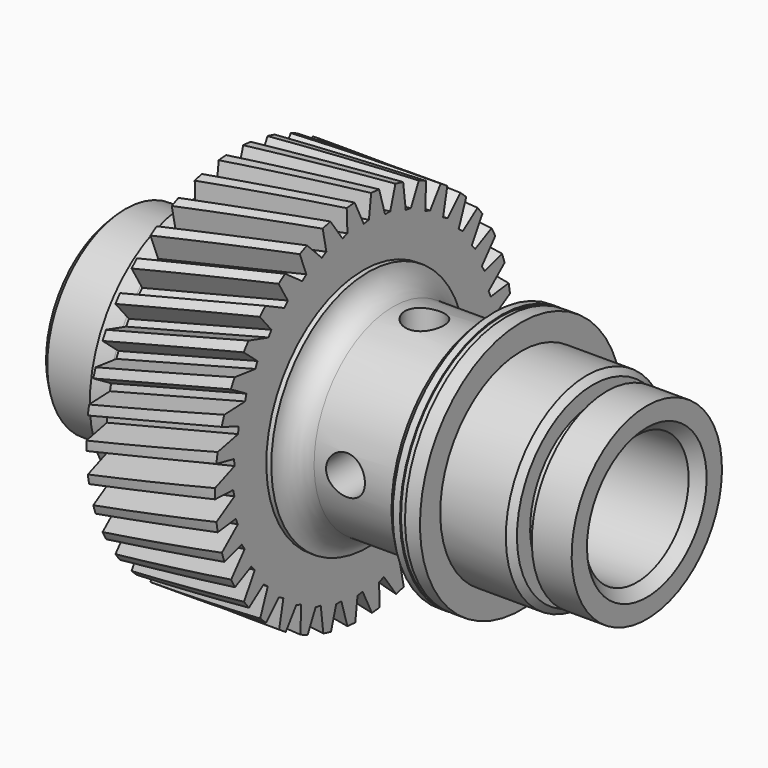
from build123d import *

# Parameters (mm, degrees)
F3_R             = 3.175
F4_SIZE          = 1.5748
F5_SIZE          = 2.54
F6_R             = 4.953
F7_DEPTH         = 47.2196
F7_DEPTH_BACK    = 47.2196
F8_R             = 4.953
F9_DEPTH         = 47.2196
F9_DEPTH_BACK    = 47.2196
F14_COPIES_COUNT = 38


# Not quite as in the source:
# - a fillet or chamfer that OpenCascade refuses, or shapes differently, is made with other operations: its cross-section is extruded or revolved along the edge and cut away or added
# - a pattern or mirror of a feature is missing from the dataset's text; its kind, count and spacing are read off the source's solid


with BuildPart() as f1:
    # F0 (on Front) → F1 (revolve)
    with BuildSketch(Plane.XZ):
        Polygon((0, 24.9174), (0, 18.6055), (28.575, 18.6055), (28.575, 13.4874), (99.4918, 13.4874), (99.4918, 16.51), (134.4168, 16.51), (134.4168, 23.9395), (124.2568, 23.9395), (124.2568, 20.0152), (120.7008, 20.0152), (120.7008, 25.7937), (102.4128, 25.7937), (102.4128, 32.258), (98.6028, 32.258), (98.6028, 31.9405), (97.3328, 31.9405), (97.3328, 32.258), (93.9038, 32.258), (93.9038, 25.146), (63.4238, 25.146), (63.4238, 30.8737), (62.1538, 30.8737), (62.1538, 47.2186), (29.3878, 47.2186), (29.3878, 32.258), (18.288, 32.258), (18.288, 24.9174), align=None)
    revolve(axis=Axis((67.2084, 0, 0), (1, 0, 0)))

    # F2: fillet of radius 6.35 on 2 edges, made by hand

    # F2_s1 → F2_t2 (revolve)
    with BuildSketch(Plane.XZ):
        with BuildLine():
            ThreePointArc((69.7432337333, 25.146), (65.4787938522, 26.7909970776), (63.4238, 30.8737))
            Line((63.4238, 30.8737), (63.4238, 25.146))
            Line((63.4238, 25.146), (69.7432337333, 25.146))
        make_face()
    revolve(axis=Axis((63.4238, 0, 0), (1, 0, 0)))

    # F2_s3 → F2_t4 (revolve)
    with BuildSketch(Plane.XZ):
        with BuildLine():
            ThreePointArc((29.3878, 38.608), (27.5279280605, 34.1178719395), (23.0378, 32.258))
            Line((23.0378, 32.258), (29.3878, 32.258))
            Line((29.3878, 32.258), (29.3878, 38.608))
        make_face()
    revolve(axis=Axis((29.3878, 0, 0), (1, 0, 0)))

    # F3
    f3_edges = [f1.edges().sort_by_distance(p)[0] for p in [
        (93.9038, 0, -25.146),
    ]]
    fillet(f3_edges, radius=F3_R)

    # F4
    f4_edges = [f1.edges().sort_by_distance(p)[0] for p in [
        (93.9038, 0, -32.258),
        (120.7008, 0, -25.7937),
        (0, 0, -24.9174),
    ]]
    chamfer(f4_edges, length=F4_SIZE)

    # F5
    f5_edges = [f1.edges().sort_by_distance(p)[0] for p in [
        (0, 0, -18.6055),
        (134.4168, 0, -16.51),
    ]]
    chamfer(f5_edges, length=F5_SIZE)

    # F6 (on Top) → F7 (cut, two sides)
    with BuildSketch(Plane.XY) as f7_sk:
        with Locations((77.7494, 0)):
            Circle(F6_R)
    extrude(amount=-F7_DEPTH, mode=Mode.SUBTRACT)
    extrude(f7_sk.sketch, amount=F7_DEPTH_BACK, mode=Mode.SUBTRACT)

    # F8 (on Front) → F9 (cut, two sides)
    with BuildSketch(Plane.XZ) as f9_sk:
        with Locations((77.7494, 0)):
            Circle(F8_R)
    extrude(amount=-F9_DEPTH, mode=Mode.SUBTRACT)
    extrude(f9_sk.sketch, amount=F9_DEPTH_BACK, mode=Mode.SUBTRACT)

    # F14: sweep along a path in F13
    with BuildLine(Plane(origin=(0.2774593378, 0, 47.3103084033), x_dir=(0.9999828033, 0, -0.005864569), z_dir=(-0.005864569, 0, -0.9999828033))) as f14_path:
        Line((29.1108412735, 2.7305), (61.8774047513, -5.0532718847))
    # F10 (on face) → F14 (sweep, cut)
    with BuildSketch(Plane(origin=(29.3878, 0, 0), x_dir=(0, -1, 0), z_dir=(-1, 0, 0))):
        with BuildLine():
            ThreePointArc((-0.8255, 40.758641277), (0, 40.767), (0.8255, 40.758641277))
            Line((0.8255, 40.758641277), (2.7305, 47.139585867))
            ThreePointArc((2.7305, 47.139585867), (0, 47.2186), (-2.7305, 47.139585867))
            Line((-2.7305, 47.139585867), (-0.8255, 40.758641277))
        make_face()
        with BuildLine():
            ThreePointArc((-2.7305, 47.139585867), (0, 47.2186), (2.7305, 47.139585867))
            Line((2.7305, 47.139585867), (3.2580456673, 48.9066408128))
            ThreePointArc((3.2580456673, 48.9066408128), (0, 49.015042356), (-3.2580456673, 48.9066408128))
            Line((-3.2580456673, 48.9066408128), (-2.7305, 47.139585867))
        make_face()
    f14 = sweep(path=f14_path.line, mode=Mode.SUBTRACT)

    # F14_copies: F14 ×38 about axis
    f14_copies_axis = Axis((0, 0, 0), (1, 0, 0))
    for i in range(1, F14_COPIES_COUNT):
        add(f14.rotate(f14_copies_axis, i * 360 / F14_COPIES_COUNT), mode=Mode.SUBTRACT)


solid = f1.part
